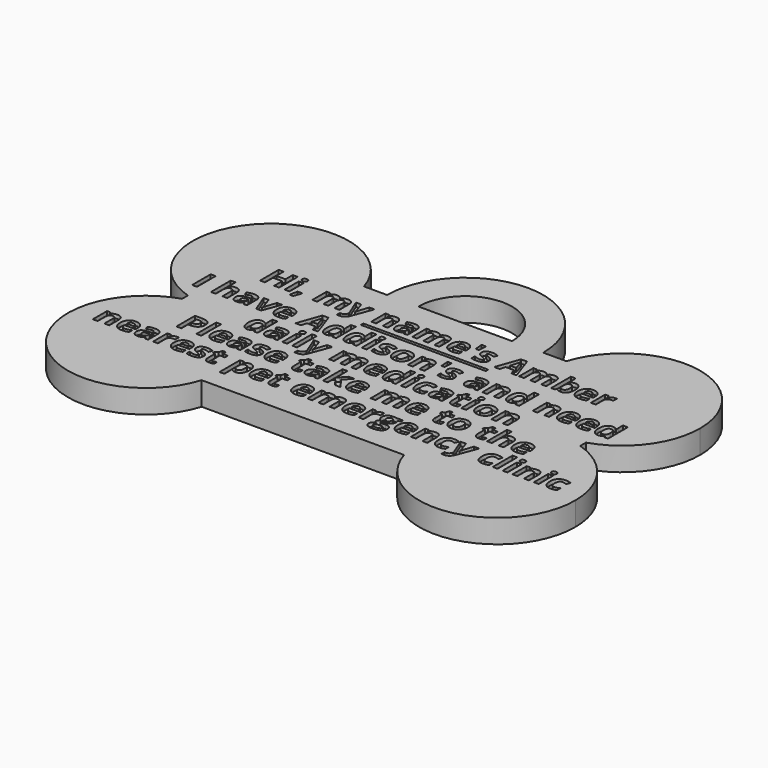
from build123d import *

# Parameters (mm, degrees)
F0_W         = 45
F0_H         = 20
F1_DEPTH     = 3
F3_DEPTH     = 3
F4_W         = 51
F4_H         = 26
F5_DEPTH     = 3
F6_R         = 10
F6_R_2       = 6
F7_DEPTH     = 3
F8_W         = 16
F8_H         = 0.4
F8_TEXT_SIZE = 4.1666666667
F9_DEPTH     = 0.5


# Not quite as in the source:
# - Text() gives the source's letters only with a copy of the font that has no kerning and outlines rounded to 1/6400 em; it was checked with that copy


with BuildPart() as f1:
    # F0 (on Top) → F1 (new body)
    with BuildSketch(Plane.XY):
        with Locations((6.4884250968, 4.8540276475)):
            Rectangle(F0_W, F0_H)
    extrude(amount=F1_DEPTH)

    # F2 (on face) → F3 (join)
    with BuildSketch(Plane.XY.offset(3)):
        with BuildLine():
            ThreePointArc((28.9884250968, 4.8540276475), (36.0594929086, 7.7829598357), (38.9884250968, 14.8540276475))
            ThreePointArc((38.9884250968, 14.8540276475), (21.9173572849, 21.9250954594), (28.9884250968, 4.8540276475))
        make_face()
        with BuildLine():
            ThreePointArc((38.9884250968, -5.1459723525), (36.0594929086, 1.9250954594), (28.9884250968, 4.8540276475))
            ThreePointArc((28.9884250968, 4.8540276475), (21.9173572849, -12.2170401643), (38.9884250968, -5.1459723525))
        make_face()
        with BuildLine():
            ThreePointArc((-16.0115749032, 4.8540276475), (-23.0826427151, -12.2170401643), (-6.0115749032, -5.1459723525))
            ThreePointArc((-6.0115749032, -5.1459723525), (-8.9405070914, 1.9250954594), (-16.0115749032, 4.8540276475))
        make_face()
        with BuildLine():
            ThreePointArc((-6.0115749032, 14.8540276475), (-23.0826427151, 21.9250954594), (-16.0115749032, 4.8540276475))
            ThreePointArc((-16.0115749032, 4.8540276475), (-8.9405070914, 7.7829598357), (-6.0115749032, 14.8540276475))
        make_face()
    extrude(amount=-F3_DEPTH)

    # F4 (on face) → F5 (join)
    with BuildSketch(Plane.XY.offset(3)):
        with Locations((6.4884250968, 4.8540276475)):
            Rectangle(F4_W, F4_H)
    extrude(amount=-F5_DEPTH)

    # F6 (on face) → F7 (join)
    with BuildSketch(Plane.XY.offset(3)):
        with Locations((6.4884250968, 17.8540276475)):
            Circle(F6_R)
        with Locations((6.4884250968, 17.8540276475)):
            Circle(F6_R_2, mode=Mode.SUBTRACT)
    extrude(amount=-F7_DEPTH)

    # F8 (on face) → F9 (cut)
    with BuildSketch(Plane.XY.offset(3)):
        with Locations((6.4884250968, 11.34627067)):
            Rectangle(F8_W, F8_H)
        with Locations((-20.4731634449, 7.3540276475)):
            Text("I have Addison's and need", F8_TEXT_SIZE, font='Open Sans', font_style=FontStyle.BOLD, text_align=(TextAlign.LEFT, TextAlign.BOTTOM))
        with Locations((-10.8244004241, 3.3540276475)):
            Text('daily medication', F8_TEXT_SIZE, font='Open Sans', font_style=FontStyle.BOLD, text_align=(TextAlign.LEFT, TextAlign.BOTTOM))
        with Locations((-16.0825384449, -0.6459723525)):
            Text('Please take me to the', F8_TEXT_SIZE, font='Open Sans', font_style=FontStyle.BOLD, text_align=(TextAlign.LEFT, TextAlign.BOTTOM))
        with Locations((-23.5395696949, -4.6459723525)):
            Text('nearest pet emergency clinic', F8_TEXT_SIZE, font='Open Sans', font_style=FontStyle.BOLD, text_align=(TextAlign.LEFT, TextAlign.BOTTOM))
        with Locations((-15.7638535491, 12.3540276475)):
            Text("Hi, my name's Amber", F8_TEXT_SIZE, font='Open Sans', font_style=FontStyle.BOLD, text_align=(TextAlign.LEFT, TextAlign.BOTTOM))
    extrude(amount=-F9_DEPTH, mode=Mode.SUBTRACT)


solid = f1.part
